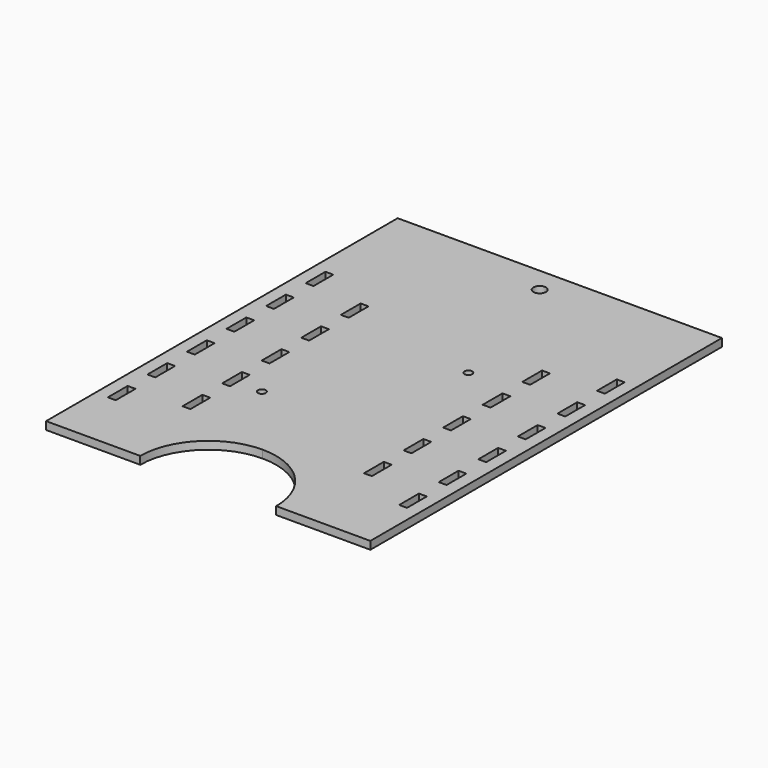
from build123d import *

# Parameters (mm, degrees)
F0_R     = 1.5875
F0_W     = 3.175
F0_H     = 10.004552
F1_DEPTH = 3.175


# Not quite as in the source:
# - a length typed as a fraction of an inch, garbled in the dataset ("3 / 203.2 mm" for 3/8 in), is restored
# - a feature names something its author has since deleted; it is built from what else it names


with BuildPart() as f1:
    # F0 (on Top) → F1 (new body)
    with BuildSketch(Plane.XY):
        with BuildLine():
            Line((-226.9615088272, -74.910188), (-188.8615088272, -74.910188))
            ThreePointArc((-188.8615088272, -74.910188), (-180.8069453098, -55.4647515174), (-161.3615088272, -47.410188))
            ThreePointArc((-161.3615088272, -47.410188), (-141.9160723446, -55.4647515174), (-133.8615088272, -74.910188))
            Line((-133.8615088272, -74.910188), (-95.7615088272, -74.910188))
            Line((-95.7615088272, -74.910188), (-95.7615088272, 102.889812))
            Line((-95.7615088272, 102.889812), (-226.9615088272, 102.889812))
            Line((-226.9615088272, 102.889812), (-226.9615088272, -74.910188))
        make_face()
        Polygon((-221.8815088272, 50.02276), (-221.8815088272, 60.027312), (-218.7065088272, 60.027312), (-218.7065088272, 50.02276), (-218.7065088272, 40.018208), (-218.7065088272, 30.013656), (-218.7065088272, 20.009104), (-218.7065088272, 10.004552), (-218.7065088272, 0), (-218.7065088272, -10.004552), (-218.7065088272, -20.009104), (-218.7065088272, -30.013656), (-218.7065088272, -40.018208), (-218.7065088272, -50.02276), (-221.8815088272, -50.02276), (-221.8815088272, -40.018208), (-221.8815088272, -30.013656), (-221.8815088272, -20.009104), (-221.8815088272, -10.004552), (-221.8815088272, 0), (-221.8815088272, 10.004552), (-221.8815088272, 20.009104), (-221.8815088272, 30.013656), (-221.8815088272, 40.018208), align=None, mode=Mode.SUBTRACT)
        Polygon((-199.6565088272, 60.027312), (-196.4815088272, 60.027312), (-196.4815088272, 50.02276), (-196.4815088272, 40.018208), (-196.4815088272, 30.013656), (-196.4815088272, 20.009104), (-196.4815088272, 10.004552), (-196.4815088272, 0), (-196.4815088272, -10.004552), (-196.4815088272, -20.009104), (-196.4815088272, -30.013656), (-196.4815088272, -40.018208), (-196.4815088272, -50.02276), (-199.6565088272, -50.02276), (-199.6565088272, -40.018208), (-199.6565088272, -30.013656), (-199.6565088272, -20.009104), (-199.6565088272, -10.004552), (-199.6565088272, 0), (-199.6565088272, 10.004552), (-199.6565088272, 20.009104), (-199.6565088272, 30.013656), (-199.6565088272, 40.018208), (-199.6565088272, 50.02276), align=None, mode=Mode.SUBTRACT)
        with Locations((-186.3334280729, -16.5444072336)):
            Circle(F0_R, mode=Mode.SUBTRACT)
        Polygon((-126.2415088272, 60.027312), (-123.0665088272, 60.027312), (-123.0665088272, 50.02276), (-123.0665088272, 40.018208), (-123.0665088272, 30.013656), (-123.0665088272, 20.009104), (-123.0665088272, 10.004552), (-123.0665088272, 0), (-123.0665088272, -10.004552), (-123.0665088272, -20.009104), (-123.0665088272, -30.013656), (-123.0665088272, -40.018208), (-123.0665088272, -50.02276), (-126.2415088272, -50.02276), (-126.2415088272, -40.018208), (-126.2415088272, -30.013656), (-126.2415088272, -20.009104), (-126.2415088272, -10.004552), (-126.2415088272, 0), (-126.2415088272, 10.004552), (-126.2415088272, 20.009104), (-126.2415088272, 30.013656), (-126.2415088272, 40.018208), (-126.2415088272, 50.02276), align=None, mode=Mode.SUBTRACT)
        Polygon((-104.0165088272, 50.02276), (-104.0165088272, 60.027312), (-100.8415088272, 60.027312), (-100.8415088272, 50.02276), (-100.8415088272, 40.018208), (-100.8415088272, 30.013656), (-100.8415088272, 20.009104), (-100.8415088272, 10.004552), (-100.8415088272, 0), (-100.8415088272, -10.004552), (-100.8415088272, -20.009104), (-100.8415088272, -30.013656), (-100.8415088272, -40.018208), (-100.8415088272, -50.02276), (-104.0165088272, -50.02276), (-104.0165088272, -40.018208), (-104.0165088272, -30.013656), (-104.0165088272, -20.009104), (-104.0165088272, -10.004552), (-104.0165088272, 0), (-104.0165088272, 10.004552), (-104.0165088272, 20.009104), (-104.0165088272, 30.013656), (-104.0165088272, 40.018208), align=None, mode=Mode.SUBTRACT)
        with BuildLine():
            ThreePointArc((-158.8215088272, 92.729812), (-159.565457603, 90.9337607758), (-161.3615088272, 90.189812))
            ThreePointArc((-161.3615088272, 90.189812), (-163.1575600514, 94.5258632242), (-158.8215088272, 92.729812))
        make_face(mode=Mode.SUBTRACT)
        with Locations((-143.4709280729, 34.2555927664)):
            Circle(F0_R, mode=Mode.SUBTRACT)
        with Locations((-198.0690088272, -45.020484)):
            Rectangle(F0_W, F0_H)
        with Locations((-198.0690088272, -25.01138)):
            Rectangle(F0_W, F0_H)
        with Locations((-198.0690088272, -5.002276)):
            Rectangle(F0_W, F0_H)
        with Locations((-198.0690088272, 15.006828)):
            Rectangle(F0_W, F0_H)
        with Locations((-198.0690088272, 35.015932)):
            Rectangle(F0_W, F0_H)
        with Locations((-198.0690088272, 55.025036)):
            Rectangle(F0_W, F0_H)
        with Locations((-220.2940088272, -35.015932)):
            Rectangle(F0_W, F0_H)
        with Locations((-220.2940088272, -15.006828)):
            Rectangle(F0_W, F0_H)
        with Locations((-220.2940088272, 5.002276)):
            Rectangle(F0_W, F0_H)
        with Locations((-220.2940088272, 25.01138)):
            Rectangle(F0_W, F0_H)
        with Locations((-220.2940088272, 45.020484)):
            Rectangle(F0_W, F0_H)
        with Locations((-102.4290088272, 45.020484)):
            Rectangle(F0_W, F0_H)
        with Locations((-102.4290088272, 25.01138)):
            Rectangle(F0_W, F0_H)
        with Locations((-102.4290088272, 5.002276)):
            Rectangle(F0_W, F0_H)
        with Locations((-102.4290088272, -15.006828)):
            Rectangle(F0_W, F0_H)
        with Locations((-102.4290088272, -35.015932)):
            Rectangle(F0_W, F0_H)
        with Locations((-124.6540088272, 55.025036)):
            Rectangle(F0_W, F0_H)
        with Locations((-124.6540088272, 35.015932)):
            Rectangle(F0_W, F0_H)
        with Locations((-124.6540088272, 15.006828)):
            Rectangle(F0_W, F0_H)
        with Locations((-124.6540088272, -5.002276)):
            Rectangle(F0_W, F0_H)
        with Locations((-124.6540088272, -25.01138)):
            Rectangle(F0_W, F0_H)
        with Locations((-124.6540088272, -45.020484)):
            Rectangle(F0_W, F0_H)
    extrude(amount=F1_DEPTH)


solid = f1.part
